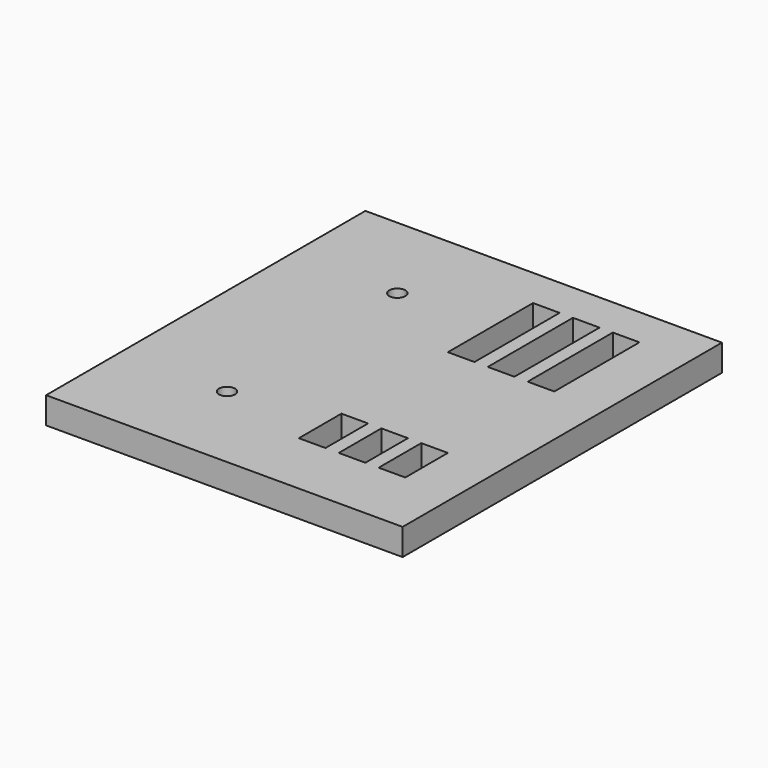
from build123d import *

# Parameters (mm, degrees)
F0_W     = 85.09
F0_H     = 95.25
F1_DEPTH = 6.35
F2_R     = 1.905
F2_W     = 6.35
F2_H     = 12.7
F2_H_2   = 6.35
F3_DEPTH = 6.351
F4_DEPTH = 132


# Not quite as in the source:
# - an extrude ends at something that could not be found from the text; its depth is read off the source's solid


with BuildPart() as f1:
    # F0 (on Top) → F1 (new body)
    with BuildSketch(Plane.XY):
        Rectangle(F0_W, F0_H)
    extrude(amount=F1_DEPTH)

    # F2 (on Top) → F3 (cut, through all)
    with BuildSketch(Plane.XY):
        with Locations((-17.145, -25.4)):
            Circle(F2_R)
        with Locations((-17.145, 25.4)):
            Circle(F2_R)
        with Locations((8.255, -25.4)):
            Rectangle(F2_W, F2_H)
        with Locations((8.255, 34.925)):
            Rectangle(F2_W, F2_H_2)
        with Locations((8.255, 25.4)):
            Rectangle(F2_W, F2_H)
        with Locations((8.255, 15.875)):
            Rectangle(F2_W, F2_H_2)
        with Locations((27.305, 25.4)):
            Rectangle(F2_W, F2_H)
        with Locations((27.305, 34.925)):
            Rectangle(F2_W, F2_H_2)
        with Locations((27.305, 15.875)):
            Rectangle(F2_W, F2_H_2)
        with Locations((27.305, -25.4)):
            Rectangle(F2_W, F2_H)
        with Locations((17.78, 34.925)):
            Rectangle(F2_W, F2_H_2)
        with Locations((17.78, 25.4)):
            Rectangle(F2_W, F2_H)
        with Locations((17.78, 15.875)):
            Rectangle(F2_W, F2_H_2)
        with Locations((17.78, -25.4)):
            Rectangle(F2_W, F2_H)
    extrude(amount=F3_DEPTH, mode=Mode.SUBTRACT)

    # F2 (on Top) → F4 (cut, through all)
    with BuildSketch(Plane.XY):
        with Locations((-17.145, -25.4)):
            Circle(F2_R)
        with Locations((-17.145, 25.4)):
            Circle(F2_R)
        with Locations((8.255, -25.4)):
            Rectangle(F2_W, F2_H)
        with Locations((8.255, 34.925)):
            Rectangle(F2_W, F2_H_2)
        with Locations((8.255, 25.4)):
            Rectangle(F2_W, F2_H)
        with Locations((8.255, 15.875)):
            Rectangle(F2_W, F2_H_2)
        with Locations((27.305, 25.4)):
            Rectangle(F2_W, F2_H)
        with Locations((27.305, 34.925)):
            Rectangle(F2_W, F2_H_2)
        with Locations((27.305, 15.875)):
            Rectangle(F2_W, F2_H_2)
        with Locations((27.305, -25.4)):
            Rectangle(F2_W, F2_H)
        with Locations((17.78, 34.925)):
            Rectangle(F2_W, F2_H_2)
        with Locations((17.78, 25.4)):
            Rectangle(F2_W, F2_H)
        with Locations((17.78, 15.875)):
            Rectangle(F2_W, F2_H_2)
        with Locations((17.78, -25.4)):
            Rectangle(F2_W, F2_H)
    extrude(amount=-F4_DEPTH, mode=Mode.SUBTRACT)


solid = f1.part
